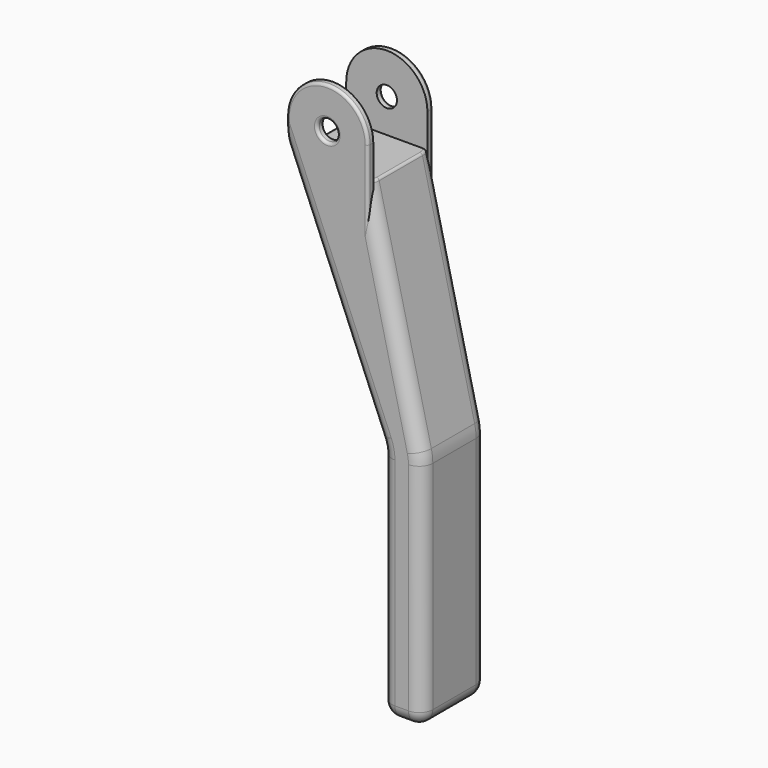
from build123d import *

# Parameters (mm, degrees)
F0_W          = 6
F0_H          = 35
F1_DEPTH      = 6
F1_DEPTH_BACK = 6
F2_DEPTH      = 6
F2_DEPTH_BACK = 6
F4_DEPTH      = 1
F6_R          = 8
F7_R          = 5
F8_T1_DEPTH   = 40.3864195747
F8_T3_DEPTH   = 8
F8_T5_DEPTH   = 2
F8_T7_DEPTH   = 31.9996073463
F8_T9_DEPTH   = 32.0603582864
F8_S13_W      = 2.04
F8_S13_H      = 2.04
F8_T14_DEPTH  = 2.04
F8_S19_W      = 2.04
F8_S19_H      = 2.04
F8_T20_DEPTH  = 2.04
F8_S25_W      = 2.04
F8_S25_H      = 2.04
F8_T26_DEPTH  = 2.04
F8_S31_W      = 2.04
F8_S31_H      = 2.04
F8_T32_DEPTH  = 2.04
F8_T38_DEPTH  = 38.5857127979
F8_T43_DEPTH  = 38.5857127979
F8_T48_DEPTH  = 38.5857127979
F8_T53_DEPTH  = 38.5857127979
F8_T56_ANGLE  = 22.6285176643
F8_T58_ANGLE  = 13.397989478
F8_T60_ANGLE  = 22.6285176643
F8_T62_ANGLE  = 13.397989478
F9_F1_R       = 0.3996
F9_F2_R       = 0.4
F9_F3_R       = 0.4
F9_F4_R       = 0.4
F9_F5_R       = 0.4
F9_F6_R       = 0.4


# Not quite as in the source:
# - a fillet or chamfer that OpenCascade refuses, or shapes differently, is made with other operations: its cross-section is extruded or revolved along the edge and cut away or added
# - a fillet or chamfer is up to 0.001 mm smaller than in the source, because OpenCascade refuses the exact size


with BuildPart() as f1:
    # F0 (on Front) → F1 (new body, two sides)
    with BuildSketch(Plane.XZ) as f1_sk:
        Polygon((12, 0), (0, 0), (14, -33.5857127979), (20, -33.5857127979), align=None)
        with Locations((17, -51.0857127979)):
            Rectangle(F0_W, F0_H)
    extrude(amount=F1_DEPTH)
    extrude(f1_sk.sketch, amount=-F1_DEPTH_BACK)

    # F0 (on Front) → F2 (join, two sides)
    with BuildSketch(Plane.XZ) as f2_sk:
        Polygon((12, 0), (0, 0), (14, -33.5857127979), (20, -33.5857127979), align=None)
        with Locations((17, -51.0857127979)):
            Rectangle(F0_W, F0_H)
    extrude(amount=F2_DEPTH)
    extrude(f2_sk.sketch, amount=-F2_DEPTH_BACK)

    # F3 (on face) → F4 (join)
    with BuildSketch(Plane.XZ.offset(6)):
        with BuildLine():
            Line((0, 5), (0, 0))
            Line((0, 0), (12, 0))
            Line((12, 0), (12, 5))
            Line((12, 5), (7.5, 5))
            ThreePointArc((7.5, 5), (6, 3.5), (4.5, 5))
            Line((4.5, 5), (0, 5))
        make_face()
        with BuildLine():
            ThreePointArc((12, 5), (6, 11), (0, 5))
            Line((0, 5), (4.5, 5))
            ThreePointArc((4.5, 5), (6, 6.5), (7.5, 5))
            Line((7.5, 5), (12, 5))
        make_face()
    extrude(amount=-F4_DEPTH)

    # F5: F1 across plane


with BuildPart() as f1_1:
    add(f1.part)
    add(f1.part.mirror(Plane.XZ))

    # F6
    f6_edges = [f1_1.edges().sort_by_distance(p)[0] for p in [
        (20, 0, -33.585713),
    ]]
    fillet(f6_edges, radius=F6_R)

    # F7
    f7_edges = [f1_1.edges().sort_by_distance(p)[0] for p in [
        (14, 0, -33.585713),
    ]]
    fillet(f7_edges, radius=F7_R)

    # F8: fillet of radius 2 on 16 edges, made by hand

    # F8_s2 → F8_t1 (cut)
    with BuildSketch(Plane(origin=(-1.9237739091, 0, 4.6150941428), x_dir=(0, 1, 0), z_dir=(0.3847547818, 0, -0.9230188286))):
        with BuildLine():
            ThreePointArc((-6, 2), (-5.4142135624, 0.5857864376), (-4, 0))
            Line((-4, 0), (-6, 0))
            Line((-6, 0), (-6, 2))
        make_face()
        with BuildLine():
            ThreePointArc((4, 0), (5.4142135624, 0.5857864376), (6, 2))
            Line((6, 2), (6, 0))
            Line((6, 0), (4, 0))
        make_face()
    extrude(amount=F8_T1_DEPTH, mode=Mode.SUBTRACT)

    # F8_s4 → F8_t3 (cut)
    with BuildSketch(Plane.XZ.offset(-4)):
        with BuildLine():
            ThreePointArc((14, -66.5857127979), (14.5857864376, -67.9999263603), (16, -68.5857127979))
            Line((16, -68.5857127979), (14, -68.5857127979))
            Line((14, -68.5857127979), (14, -66.5857127979))
        make_face()
        with BuildLine():
            ThreePointArc((18, -68.5857127979), (19.4142135624, -67.9999263603), (20, -66.5857127979))
            Line((20, -66.5857127979), (20, -68.5857127979))
            Line((20, -68.5857127979), (18, -68.5857127979))
        make_face()
    extrude(amount=F8_T3_DEPTH, mode=Mode.SUBTRACT)

    # F8_s6 → F8_t5 (cut)
    with BuildSketch(Plane.YZ.offset(16)):
        with BuildLine():
            ThreePointArc((-6, -66.5857127979), (-5.4142135624, -67.9999263603), (-4, -68.5857127979))
            Line((-4, -68.5857127979), (-6, -68.5857127979))
            Line((-6, -68.5857127979), (-6, -66.5857127979))
        make_face()
        with BuildLine():
            ThreePointArc((4, -68.5857127979), (5.4142135624, -67.9999263603), (6, -66.5857127979))
            Line((6, -66.5857127979), (6, -68.5857127979))
            Line((6, -68.5857127979), (4, -68.5857127979))
        make_face()
    extrude(amount=F8_T5_DEPTH, mode=Mode.SUBTRACT)

    # F8_s8 → F8_t7 (cut)
    with BuildSketch(Plane.XY.offset(-66.5857127979)):
        with BuildLine():
            ThreePointArc((16, -6), (14.5857864376, -5.4142135624), (14, -4))
            Line((14, -4), (14, -6))
            Line((14, -6), (16, -6))
        make_face()
        with BuildLine():
            ThreePointArc((14, 4), (14.5857864376, 5.4142135624), (16, 6))
            Line((16, 6), (14, 6))
            Line((14, 6), (14, 4))
        make_face()
    extrude(amount=F8_T7_DEPTH, mode=Mode.SUBTRACT)

    # F8_s10 → F8_t9 (cut)
    with BuildSketch(Plane.XY.offset(-66.5857127979)):
        with BuildLine():
            ThreePointArc((18, -6), (19.4142135624, -5.4142135624), (20, -4))
            Line((20, -4), (20, -6))
            Line((20, -6), (18, -6))
        make_face()
        with BuildLine():
            ThreePointArc((20, 4), (19.4142135624, 5.4142135624), (18, 6))
            Line((18, 6), (20, 6))
            Line((20, 6), (20, 4))
        make_face()
    extrude(amount=F8_T9_DEPTH, mode=Mode.SUBTRACT)


with BuildPart() as f8_tool12:
    # F8_s13 → F8_t14 (new body)
    with BuildSketch(Plane.XZ.offset(4)):
        with Locations((14.98, -67.6057127979)):
            Rectangle(F8_S13_W, F8_S13_H)
    extrude(amount=F8_T14_DEPTH)

    # F8_s15 → F8_t16 (revolve, cut)
    with BuildSketch(Plane(origin=(16, -4, -66.5857127979), x_dir=(0.7071067812, 0, 0.7071067812), z_dir=(0.7071067812, 0, -0.7071067812))):
        with BuildLine():
            ThreePointArc((0, -2), (2, 0), (0, 2))
            Line((0, 2), (0, -2))
        make_face()
    revolve(axis=Axis((16, -4, -66.5857127979), (0, -1, 0)), mode=Mode.SUBTRACT)


with BuildPart() as f1_2:
    add(f1_1.part)

    # F8_t11: cut F8_tool12
    add(f8_tool12.part, mode=Mode.SUBTRACT)


with BuildPart() as f8_tool18:
    # F8_s19 → F8_t20 (new body)
    with BuildSketch(Plane.YZ.offset(16)):
        with Locations((5.02, -67.6057127979)):
            Rectangle(F8_S19_W, F8_S19_H)
    extrude(amount=-F8_T20_DEPTH)

    # F8_s21 → F8_t22 (revolve, cut)
    with BuildSketch(Plane(origin=(16, 4, -66.5857127979), x_dir=(0, -0.7071067812, 0.7071067812), z_dir=(0, -0.7071067812, -0.7071067812))):
        with BuildLine():
            ThreePointArc((0, -2), (2, 0), (0, 2))
            Line((0, 2), (0, -2))
        make_face()
    revolve(axis=Axis((16, 4, -66.5857127979), (-1, 0, 0)), mode=Mode.SUBTRACT)


with BuildPart() as f1_3:
    add(f1_2.part)

    # F8_t17: cut F8_tool18
    add(f8_tool18.part, mode=Mode.SUBTRACT)


with BuildPart() as f8_tool24:
    # F8_s25 → F8_t26 (new body)
    with BuildSketch(Plane.XZ.offset(4)):
        with Locations((19.02, -67.6057127979)):
            Rectangle(F8_S25_W, F8_S25_H)
    extrude(amount=F8_T26_DEPTH)

    # F8_s27 → F8_t28 (revolve, cut)
    with BuildSketch(Plane(origin=(18, -4, -66.5857127979), x_dir=(-0.7071067812, 0, 0.7071067812), z_dir=(0.7071067812, 0, 0.7071067812))):
        with BuildLine():
            ThreePointArc((0, -2), (2, 0), (0, 2))
            Line((0, 2), (0, -2))
        make_face()
    revolve(axis=Axis((18, -4, -66.5857127979), (0, -1, 0)), mode=Mode.SUBTRACT)


with BuildPart() as f1_4:
    add(f1_3.part)

    # F8_t23: cut F8_tool24
    add(f8_tool24.part, mode=Mode.SUBTRACT)


with BuildPart() as f8_tool30:
    # F8_s31 → F8_t32 (new body)
    with BuildSketch(Plane.XY.offset(-66.5857127979)):
        with Locations((19.02, 5.02)):
            Rectangle(F8_S31_W, F8_S31_H)
    extrude(amount=-F8_T32_DEPTH)

    # F8_s33 → F8_t34 (revolve, cut)
    with BuildSketch(Plane(origin=(18, 4, -66.5857127979), x_dir=(-0.7071067812, -0.7071067812, 0), z_dir=(0.7071067812, -0.7071067812, 0))):
        with BuildLine():
            ThreePointArc((0, -2), (2, 0), (0, 2))
            Line((0, 2), (0, -2))
        make_face()
    revolve(axis=Axis((18, 4, -66.5857127979), (0, 0, -1)), mode=Mode.SUBTRACT)


with BuildPart() as f1_5:
    add(f1_4.part)

    # F8_t29: cut F8_tool30
    add(f8_tool30.part, mode=Mode.SUBTRACT)


with BuildPart() as f8_tool36:
    # F8_s37 → F8_t38 (new body)
    with BuildSketch(Plane(origin=(8.4265673233, 0, -35.3765337491), x_dir=(0, 1, 0), z_dir=(-0.2317137684, 0, 0.9727840097))):
        with BuildLine():
            ThreePointArc((-6, -9.6734081164), (-5.4142135624, -11.0876216787), (-4, -11.6734081164))
            Line((-4, -11.6734081164), (-6, -11.6734081164))
            Line((-6, -11.6734081164), (-6, -9.6734081164))
        make_face()
    extrude(amount=F8_T38_DEPTH)

    split(bisect_by=Plane.YZ.offset(12), keep=Keep.TOP)


with BuildPart() as f1_6:
    add(f1_5.part)

    # F8_t35: cut F8_tool36
    add(f8_tool36.part, mode=Mode.SUBTRACT)


with BuildPart() as f8_tool41:
    # F8_s42 → F8_t43 (new body)
    with BuildSketch(Plane(origin=(8.4265673233, 0, -35.3765337491), x_dir=(0, 1, 0), z_dir=(-0.2317137684, 0, 0.9727840097))):
        with BuildLine():
            ThreePointArc((-6, -9.6734081164), (-5.4142135624, -11.0876216787), (-4, -11.6734081164))
            Line((-4, -11.6734081164), (-6, -11.6734081164))
            Line((-6, -11.6734081164), (-6, -9.6734081164))
        make_face()
    extrude(amount=F8_T43_DEPTH)

    split(bisect_by=Plane.XZ.offset(5), keep=Keep.BOTTOM)


with BuildPart() as f1_7:
    add(f1_6.part)

    # F8_t40: cut F8_tool41
    add(f8_tool41.part, mode=Mode.SUBTRACT)


with BuildPart() as f8_tool46:
    # F8_s47 → F8_t48 (new body)
    with BuildSketch(Plane(origin=(8.4265673233, 0, -35.3765337491), x_dir=(0, 1, 0), z_dir=(-0.2317137684, 0, 0.9727840097))):
        with BuildLine():
            ThreePointArc((4, -11.6734081164), (5.4142135624, -11.0876216787), (6, -9.6734081164))
            Line((6, -9.6734081164), (6, -11.6734081164))
            Line((6, -11.6734081164), (4, -11.6734081164))
        make_face()
    extrude(amount=F8_T48_DEPTH)

    split(bisect_by=Plane.YZ.offset(12), keep=Keep.TOP)


with BuildPart() as f1_8:
    add(f1_7.part)

    # F8_t45: cut F8_tool46
    add(f8_tool46.part, mode=Mode.SUBTRACT)


with BuildPart() as f8_tool51:
    # F8_s52 → F8_t53 (new body)
    with BuildSketch(Plane(origin=(8.4265673233, 0, -35.3765337491), x_dir=(0, 1, 0), z_dir=(-0.2317137684, 0, 0.9727840097))):
        with BuildLine():
            ThreePointArc((4, -11.6734081164), (5.4142135624, -11.0876216787), (6, -9.6734081164))
            Line((6, -9.6734081164), (6, -11.6734081164))
            Line((6, -11.6734081164), (4, -11.6734081164))
        make_face()
    extrude(amount=F8_T53_DEPTH)

    split(bisect_by=Plane.XZ.offset(-5), keep=Keep.TOP)


with BuildPart() as f1_9:
    add(f1_8.part)

    # F8_t50: cut F8_tool51
    add(f8_tool51.part, mode=Mode.SUBTRACT)

    # F8_s55 → F8_t56 (revolve, cut)
    with BuildSketch(Plane.XY.offset(-34.5861054517)):
        with BuildLine():
            ThreePointArc((16, -6), (14.5857864376, -5.4142135624), (14, -4))
            Line((14, -4), (14, -6))
            Line((14, -6), (16, -6))
        make_face()
    revolve(axis=Axis((9, -6, -34.5861054517), (0, -1, 0)), revolution_arc=F8_T56_ANGLE, mode=Mode.SUBTRACT)

    # F8_s57 → F8_t58 (revolve, cut)
    with BuildSketch(Plane(origin=(8.4265673233, 0, -35.3765337491), x_dir=(0, 1, 0), z_dir=(-0.2317137684, 0, 0.9727840097))):
        with BuildLine():
            ThreePointArc((-6, -9.6734081164), (-5.4142135624, -11.0876216787), (-4, -11.6734081164))
            Line((-4, -11.6734081164), (-6, -11.6734081164))
            Line((-6, -11.6734081164), (-6, -9.6734081164))
        make_face()
    revolve(axis=Axis((12, -6, -34.5253545115), (0, 1, 0)), revolution_arc=F8_T58_ANGLE, mode=Mode.SUBTRACT)

    # F8_s59 → F8_t60 (revolve, cut)
    with BuildSketch(Plane.XY.offset(-34.5861054517)):
        with BuildLine():
            ThreePointArc((14, 4), (14.5857864376, 5.4142135624), (16, 6))
            Line((16, 6), (14, 6))
            Line((14, 6), (14, 4))
        make_face()
    revolve(axis=Axis((9, 6, -34.5861054517), (0, -1, 0)), revolution_arc=F8_T60_ANGLE, mode=Mode.SUBTRACT)

    # F8_s61 → F8_t62 (revolve, cut)
    with BuildSketch(Plane(origin=(8.4265673233, 0, -35.3765337491), x_dir=(0, 1, 0), z_dir=(-0.2317137684, 0, 0.9727840097))):
        with BuildLine():
            ThreePointArc((4, -11.6734081164), (5.4142135624, -11.0876216787), (6, -9.6734081164))
            Line((6, -9.6734081164), (6, -11.6734081164))
            Line((6, -11.6734081164), (4, -11.6734081164))
        make_face()
    revolve(axis=Axis((12, 6, -34.5253545115), (0, 1, 0)), revolution_arc=F8_T62_ANGLE, mode=Mode.SUBTRACT)

    # F9: fillet of radius 0.4 on 14 edges, made by hand

    # F9_f1 (radius 0.4 in the source; OpenCascade refuses exactly that, so slightly less here)
    f9_f1_edges = [f1_9.edges().sort_by_distance(p)[0] for p in [
        (6.0954289614, -6, 10.9992410614),
        (12, -6, -1.8156693139),
        (0.0007571531, -5.9996225622, 5.095316653),
        (0, -5.7126761816, 2.5137278107),
    ]]
    fillet(f9_f1_edges, radius=F9_F1_R)

    # F9_f2
    f9_f2_edges = [f1_9.edges().sort_by_distance(p)[0] for p in [
        (7.5, -6, 5),
    ]]
    fillet(f9_f2_edges, radius=F9_F2_R)

    # F9_f3
    f9_f3_edges = [f1_9.edges().sort_by_distance(p)[0] for p in [
        (0.073832023, -4.5176380902, 0),
        (0, 0, 0),
        (0.073832023, 4.5176380902, 0),
    ]]
    fillet(f9_f3_edges, radius=F9_F3_R)

    # F9_f4
    f9_f4_edges = [f1_9.edges().sort_by_distance(p)[0] for p in [
        (11.9299450374, -4.5176380902, 0),
        (12, 0, 0),
        (11.9299450374, 4.5176380902, 0),
    ]]
    fillet(f9_f4_edges, radius=F9_F4_R)

    # F9_f5
    f9_f5_edges = [f1_9.edges().sort_by_distance(p)[0] for p in [
        (0, 5.7126761816, 2.5137278107),
        (0.0007571531, 5.9996225621, 5.0953166531),
        (6.0954289614, 6, 10.9992410614),
        (12, 6, -1.8156693139),
    ]]
    fillet(f9_f5_edges, radius=F9_F5_R)

    # F9_f6
    f9_f6_edges = [f1_9.edges().sort_by_distance(p)[0] for p in [
        (7.5, 6, 5),
    ]]
    fillet(f9_f6_edges, radius=F9_F6_R)


solid = f1_9.part
